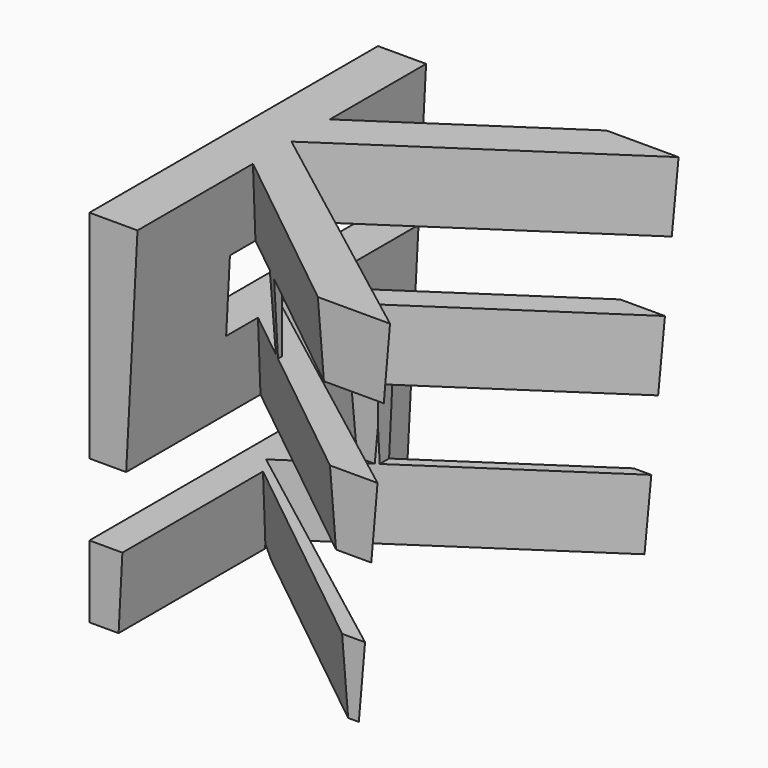
from build123d import *

# Parameters (mm, degrees)
F0_W                      = 38.1
F0_H                      = 38.0999962341
F1_DEPTH                  = 38.1
F5_W                      = 25.4
F5_H                      = 7.62
F6_DEPTH                  = 38.1
F7_W                      = 27.94
F7_H                      = 7.62
F8_DEPTH                  = 38.1
F10_DEPTH                 = 38.1
DRAFT_F10_DRAFTED_ANGLE   = -3
DRAFT_F10_2_DRAFTED_ANGLE = -3
DRAFT_F10_3_DRAFTED_ANGLE = -3


# Not quite as in the source:
# - an extrude with a draft is written as a straight extrude whose walls are then drafted


with BuildPart() as f1:
    # F0 (on Front) → F1 (new body)
    with BuildSketch(Plane.XZ):
        with Locations((19.05, 19.049998117)):
            Rectangle(F0_W, F0_H)
    extrude(amount=F1_DEPTH)

    # F5 (on offset) → F6 (cut)
    with BuildSketch(Plane.YZ.offset(38.1)):
        with Locations((-12.7, 26.67)):
            Rectangle(F5_W, F5_H)
        with Locations((-25.4, 11.43)):
            Rectangle(F5_W, F5_H)
    extrude(amount=-F6_DEPTH, mode=Mode.SUBTRACT)

    # F7 (on offset) → F8 (cut)
    with BuildSketch(Plane.XZ.offset(38.1)):
        with Locations((24.13, 26.67)):
            Rectangle(F7_W, F7_H)
        with Locations((24.13, 11.43)):
            Rectangle(F7_W, F7_H)
    extrude(amount=-F8_DEPTH, mode=Mode.SUBTRACT)


with BuildPart() as f10_drafted:
    # F9 (on offset) → F10 (new body)
    with BuildSketch(Plane.XY.offset(38.1)):
        Polygon((5.08, -22.86), (5.08, -38.1), (24.13, -38.1), align=None)
    extrude(amount=-F10_DEPTH)

    # draft_F10_drafted
    draft_f10_drafted_walls = [f10_drafted.faces().sort_by_distance(p)[0] for p in [
        (14.605, -30.48, 12.7),
        (5.08, -30.48, 12.7),
        (14.605, -38.1, 12.7),
    ]]
    draft(draft_f10_drafted_walls, neutral_plane=Plane(origin=(0, 0, 38.1), x_dir=(1, 0, 0), z_dir=(0, 0, -1)), angle=DRAFT_F10_DRAFTED_ANGLE)


with BuildPart() as f1_1:
    add(f1.part)

    # join_F10_drafted: cut F10_drafted
    add(f10_drafted.part, mode=Mode.SUBTRACT)


with BuildPart() as f10_2_drafted:
    # F9 (on offset) → F10, piece 2 (new body)
    with BuildSketch(Plane.XY.offset(38.1)):
        Polygon((38.1, 0), (31.75, 0), (5.08, -17.78), (31.75, -38.1), (38.1, -38.1), align=None)
    extrude(amount=-F10_DEPTH)

    # draft_F10_2_drafted
    draft_f10_2_drafted_walls = [f10_2_drafted.faces().sort_by_distance(p)[0] for p in [
        (34.925, 0, 12.7),
        (18.415, -8.89, 12.7),
        (18.415, -27.94, 12.7),
        (34.925, -38.1, 12.7),
        (38.1, -19.05, 12.7),
    ]]
    draft(draft_f10_2_drafted_walls, neutral_plane=Plane(origin=(0, 0, 38.1), x_dir=(1, 0, 0), z_dir=(0, 0, -1)), angle=DRAFT_F10_2_DRAFTED_ANGLE)


with BuildPart() as f1_2:
    add(f1_1.part)

    # join_F10_2_drafted: cut F10_2_drafted
    add(f10_2_drafted.part, mode=Mode.SUBTRACT)


with BuildPart() as f10_3_drafted:
    # F9 (on offset) → F10, piece 3 (new body)
    with BuildSketch(Plane.XY.offset(38.1)):
        Polygon((24.13, 0), (5.08, 0), (5.08, -12.7), align=None)
    extrude(amount=-F10_DEPTH)

    # draft_F10_3_drafted
    draft_f10_3_drafted_walls = [f10_3_drafted.faces().sort_by_distance(p)[0] for p in [
        (14.605, 0, 12.7),
        (5.08, -6.35, 12.7),
        (14.605, -6.35, 12.7),
    ]]
    draft(draft_f10_3_drafted_walls, neutral_plane=Plane(origin=(0, 0, 38.1), x_dir=(1, 0, 0), z_dir=(0, 0, -1)), angle=DRAFT_F10_3_DRAFTED_ANGLE)


with BuildPart() as f1_3:
    add(f1_2.part)

    # join_F10_3_drafted: cut F10_3_drafted
    add(f10_3_drafted.part, mode=Mode.SUBTRACT)


solid = f1_3.part
